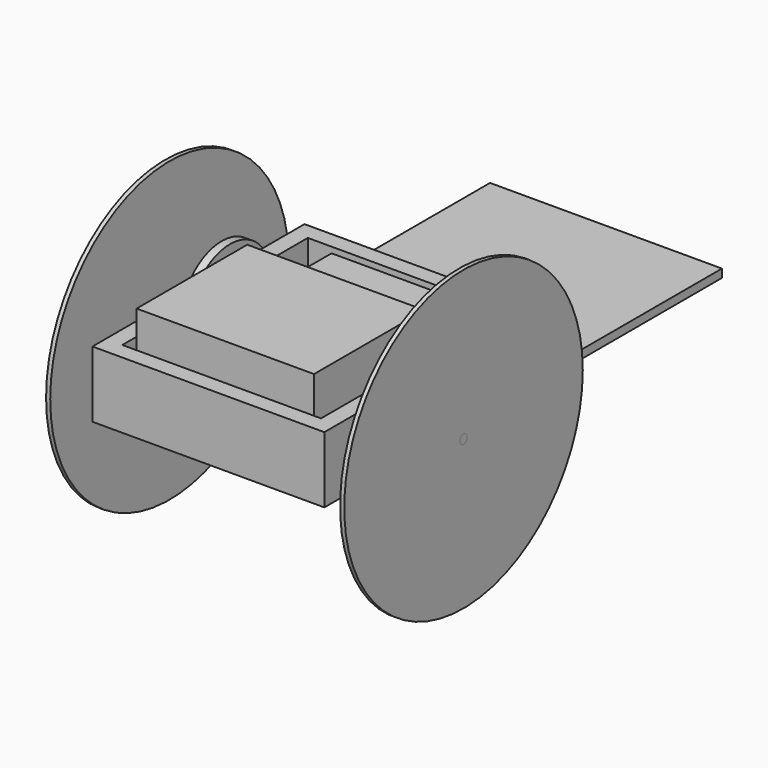
from build123d import *

# Parameters (mm, degrees)
F0_W           = 88.9
F0_H           = 101.6
F0_W_2         = 76.2
F0_H_2         = 88.9
F1_DEPTH       = 25.4
F2_DEPTH       = 3.175
F3_W           = 88.9
F3_H           = 3.175
F4_DEPTH       = 76.2
F5_W           = 47.999904
F5_H           = 25.0000008
F6_DEPTH       = 15.0114
F5_W_2         = 68.000118
F5_H_2         = 52.999894
F7_DEPTH       = 26.0096
F8_R           = 1.7859375
F9_DEPTH       = 6.35
F10_R          = 1.7859375
F11_DEPTH      = 6.35
F12_DEPTH      = 57.15
F12_DEPTH_BACK = 57.15
F15_R          = 57.15
F15_R_2        = 1.7859375
F16_DEPTH      = 1.5875
F17_R          = 57.15
F17_R_2        = 1.7859375
F18_DEPTH      = 1.5875
F20_R          = 1.7859375
F21_DEPTH      = 3.175
F22_R          = 5.0000027
F22_R_2        = 1.7859375
F23_DEPTH      = 3.175
F20_R_2        = 19.99996
F24_DEPTH      = 3.175
F25_DEPTH      = 3.175
F26_DEPTH      = 3.175
F27_W          = 22
F27_H          = 21
F28_DEPTH      = 12


# Not quite as in the source:
# - a length typed as a fraction of an inch, garbled in the dataset ("3 / 203.2 mm" for 3/8 in), is restored


with BuildPart() as f1:
    # F0 (on Top) → F1 (new body)
    with BuildSketch(Plane.XY):
        Rectangle(F0_W, F0_H)
        Rectangle(F0_W_2, F0_H_2, mode=Mode.SUBTRACT)
    extrude(amount=F1_DEPTH)

    # F0 (on Top) → F2 (join)
    with BuildSketch(Plane.XY):
        Rectangle(F0_W_2, F0_H_2)
    extrude(amount=F2_DEPTH)

    # F8 (on face) → F9 (cut)
    with BuildSketch(Plane(origin=(-44.45, 0, 0), x_dir=(0, -1, 0), z_dir=(-1, 0, 0))):
        with Locations((0, 6.5484375)):
            Circle(F8_R)
    extrude(amount=-F9_DEPTH, mode=Mode.SUBTRACT)

    # F10 (on face) → F11 (cut)
    with BuildSketch(Plane.YZ.offset(44.45)):
        with Locations((0, 6.5484375)):
            Circle(F10_R)
    extrude(amount=-F11_DEPTH, mode=Mode.SUBTRACT)

    # F0 (on Top) → F26 (join)
    with BuildSketch(Plane.XY):
        with Locations((0, 95.25)):
            Rectangle(F0_W, F0_H_2)
    extrude(amount=F26_DEPTH)


with BuildPart() as f4:
    # F3 (on face) → F4 (new body)
    with BuildSketch(Plane.YZ.offset(-38.1)):
        with Locations((0, 10.715625)):
            Rectangle(F3_W, F3_H)
    extrude(amount=F4_DEPTH)


with BuildPart() as f6:
    # F5 (on face) → F6 (new body)
    with BuildSketch(Plane.XY.offset(12.303125)):
        with Locations((0, 25.7093309629)):
            Rectangle(F5_W, F5_H)
    extrude(amount=F6_DEPTH)


with BuildPart() as f7:
    # F5 (on face) → F7 (new body)
    with BuildSketch(Plane.XY.offset(12.303125)):
        with Locations((0, -16.2006690371)):
            Rectangle(F5_W_2, F5_H_2)
    extrude(amount=F7_DEPTH)


with BuildPart() as f12:
    # F8 (on face) → F12 (new body, two sides)
    with BuildSketch(Plane(origin=(-44.45, 0, 0), x_dir=(0, -1, 0), z_dir=(-1, 0, 0))) as f12_sk:
        with Locations((0, 6.5484375)):
            Circle(F8_R)
    extrude(amount=-F12_DEPTH)
    extrude(f12_sk.sketch, amount=F12_DEPTH_BACK)


with BuildPart() as f12_1:
    # F13: moved
    add(f12.part.moved(Location((38.1, 0, 0))))


with BuildPart() as f12_2:
    # F14: moved
    add(f12_1.part.moved(Location((6.35, 0, 0))))


with BuildPart() as f16:
    # F15 (on face) → F16 (new body)
    with BuildSketch(Plane.YZ.offset(57.15)):
        with Locations((0, 6.5484375)):
            Circle(F15_R)
        with Locations((0, 6.5484375)):
            Circle(F15_R_2, mode=Mode.SUBTRACT)
    extrude(amount=-F16_DEPTH)


with BuildPart() as f18:
    # F17 (on face) → F18 (new body)
    with BuildSketch(Plane(origin=(-57.15, 0, 0), x_dir=(0, -1, 0), z_dir=(-1, 0, 0))):
        with Locations((0, 6.5484375)):
            Circle(F17_R)
        with Locations((0, 6.5484375)):
            Circle(F17_R_2, mode=Mode.SUBTRACT)
    extrude(amount=-F18_DEPTH)


with BuildPart() as f21:
    # F20 (on face) → F21 (new body)
    with BuildSketch(Plane(origin=(55.5625, 0, 0), x_dir=(0, -1, 0), z_dir=(-1, 0, 0))):
        with BuildLine():
            ThreePointArc((-5.0000027, 6.5484375), (0, 1.5484348), (5.0000027, 6.5484375))
            ThreePointArc((5.0000027, 6.5484375), (0, 11.5484402), (-5.0000027, 6.5484375))
        make_face()
        with Locations((0, 6.5484375)):
            Circle(F20_R, mode=Mode.SUBTRACT)
    extrude(amount=F21_DEPTH)


with BuildPart() as f23:
    # F22 (on face) → F23 (new body)
    with BuildSketch(Plane.YZ.offset(-55.5625)):
        with Locations((0, 6.5484375)):
            Circle(F22_R)
        with Locations((0, 6.5484375)):
            Circle(F22_R_2, mode=Mode.SUBTRACT)
    extrude(amount=F23_DEPTH)


with BuildPart() as f24:
    # F20 (on face) → F24 (new body)
    with BuildSketch(Plane(origin=(55.5625, 0, 0), x_dir=(0, -1, 0), z_dir=(-1, 0, 0))):
        with Locations((-24.9999627, 6.5484375)):
            Circle(F20_R_2)
    extrude(amount=F24_DEPTH)


with BuildPart() as f25:
    # F22 (on face) → F25 (new body)
    with BuildSketch(Plane.YZ.offset(-55.5625)):
        with BuildLine():
            ThreePointArc((44.9999227, 6.5484375), (24.9999627, 26.5483975), (5.0000027, 6.5484375))
            ThreePointArc((5.0000027, 6.5484375), (24.9999627, -13.4515225), (44.9999227, 6.5484375))
        make_face()
    extrude(amount=F25_DEPTH)


with BuildPart() as f28:
    # F27 (on face) → F28 (new body)
    with BuildSketch(Plane(origin=(0, 0, 0), x_dir=(1, 0, 0), z_dir=(0, 0, -1))):
        with Locations((-33.45, -25)):
            Rectangle(F27_W, F27_H)
    extrude(amount=F28_DEPTH)


with BuildPart() as f28b:
    # F27 (on face) → F28, piece 2 (new body)
    with BuildSketch(Plane(origin=(0, 0, 0), x_dir=(1, 0, 0), z_dir=(0, 0, -1))):
        with Locations((33.45, -25)):
            Rectangle(F27_W, F27_H)
    extrude(amount=F28_DEPTH)


solid = Compound([f1.part, f4.part, f6.part, f7.part, f12_2.part, f16.part, f18.part, f21.part, f23.part, f24.part, f25.part, f28.part, f28b.part])
